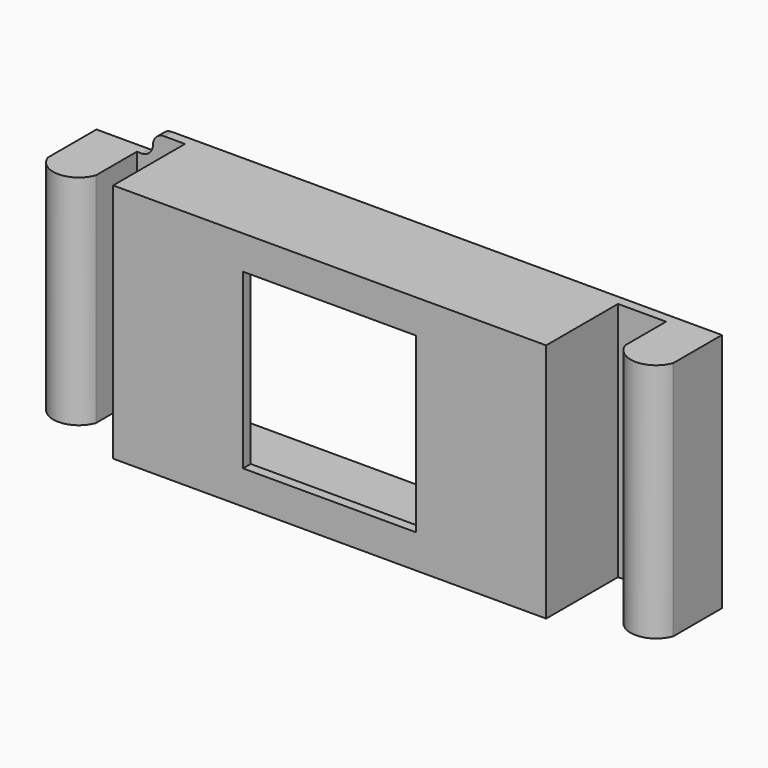
from build123d import *

# Parameters (mm, degrees)
F0_W      = 60
F0_H      = 60
F0_R      = 22.4096796893
F1_DEPTH  = 3
F2_W      = 60
F2_H      = 60
F2_W_2    = 54
F2_H_2    = 54
F3_DEPTH  = 15
F4_W      = 135
F4_H      = 75
F4_W_2    = 54
F4_H_2    = 54
F5_DEPTH  = 3
F6_W      = 135
F6_H      = 75
F6_W_2    = 129
F6_H_2    = 69
F7_DEPTH  = 25
F8_W      = 195
F8_H      = 75
F8_W_2    = 129
F8_H_2    = 69
F9_DEPTH  = 3
F10_W     = 15
F10_H     = 68
F11_DEPTH = 25
F12_W     = 15
F12_H     = 75
F13_DEPTH = 25
F15_DEPTH = 200
F17_DEPTH = 25
F18_R     = 3.49999
F21_DEPTH = 60
F24_W     = 60
F24_H     = 60
F25_DEPTH = 18


# Not quite as in the source:
# - a fillet or chamfer is up to 0.001 mm smaller than in the source, because OpenCascade refuses the exact size


with BuildPart() as f1:
    # F0 (on Front) → F1 (new body)
    with BuildSketch(Plane.XZ):
        Rectangle(F0_W, F0_H)
        Circle(F0_R, mode=Mode.SUBTRACT)
    extrude(amount=F1_DEPTH)

    # F2 (on face) → F3 (join)
    with BuildSketch(Plane(origin=(0, 0, 0), x_dir=(-1, 0, 0), z_dir=(0, 1, 0))):
        Rectangle(F2_W, F2_H)
        Rectangle(F2_W_2, F2_H_2, mode=Mode.SUBTRACT)
    extrude(amount=F3_DEPTH)

    # F4 (on face) → F5 (join)
    with BuildSketch(Plane(origin=(0, 15, 0), x_dir=(-1, 0, 0), z_dir=(0, 1, 0))):
        Rectangle(F4_W, F4_H)
        Rectangle(F4_W_2, F4_H_2, mode=Mode.SUBTRACT)
    extrude(amount=F5_DEPTH)

    # F6 (on face) → F7 (join)
    with BuildSketch(Plane(origin=(0, 18, 0), x_dir=(-1, 0, 0), z_dir=(0, 1, 0))):
        Rectangle(F6_W, F6_H)
        Rectangle(F6_W_2, F6_H_2, mode=Mode.SUBTRACT)
    extrude(amount=F7_DEPTH)

    # F8 (on face) → F9 (join)
    with BuildSketch(Plane(origin=(0, 43, 0), x_dir=(-1, 0, 0), z_dir=(0, 1, 0))):
        Rectangle(F8_W, F8_H)
        Rectangle(F8_W_2, F8_H_2, mode=Mode.SUBTRACT)
    extrude(amount=F9_DEPTH)

    # F10 (on face) → F11 (join)
    with BuildSketch(Plane.XZ.offset(-43)):
        with Locations((-90, -3.5)):
            Rectangle(F10_W, F10_H)
    extrude(amount=F11_DEPTH)

    # F12 (on face) → F13 (join)
    with BuildSketch(Plane.XZ.offset(-43)):
        with Locations((90, 0)):
            Rectangle(F12_W, F12_H)
    extrude(amount=F13_DEPTH)

    # F14 (on face) → F15 (cut)
    with BuildSketch(Plane.XY.offset(37.5)):
        with BuildLine():
            ThreePointArc((-82.5, 27), (-90, 21.7838821814), (-97.5, 27))
            Line((-97.5, 27), (-97.5, 18))
            Line((-97.5, 18), (-82.5, 18))
            Line((-82.5, 18), (-82.5, 27))
        make_face()
        with BuildLine():
            ThreePointArc((97.5, 27), (90, 21.7838821814), (82.5, 27))
            Line((82.5, 27), (82.5, 18))
            Line((82.5, 18), (97.5, 18))
            Line((97.5, 18), (97.5, 27))
        make_face()
    extrude(amount=-F15_DEPTH, mode=Mode.SUBTRACT)

    # F16 (on face) → F17 (cut)
    with BuildSketch(Plane.XZ.offset(-43)):
        Polygon((-77.5, 37.5), (-82.5, 37.5), (-97.5, 37.5), (-97.5, 30.5), (-82.5, 30.5), (-77.5, 30.5), align=None)
    extrude(amount=-F17_DEPTH, mode=Mode.SUBTRACT)

    # F18 (radius 3.5 in the source; OpenCascade refuses exactly that, so slightly less here)
    f18_edges = [f1.edges().sort_by_distance(p)[0] for p in [
        (-77.5, 44.5, 30.5),
        (-77.5, 44.5, 37.5),
    ]]
    fillet(f18_edges, radius=F18_R)

    # F20 (on face) → F21 (cut)
    with BuildSketch(Plane.XY.offset(30)):
        Polygon((-30, -3), (-50, 15), (-50, -3), align=None)
    extrude(amount=-F21_DEPTH, mode=Mode.SUBTRACT)

    # F24 (on face) → F25 (cut)
    with BuildSketch(Plane.XZ.offset(3)):
        Rectangle(F24_W, F24_H)
    extrude(amount=-F25_DEPTH, mode=Mode.SUBTRACT)


solid = f1.part
